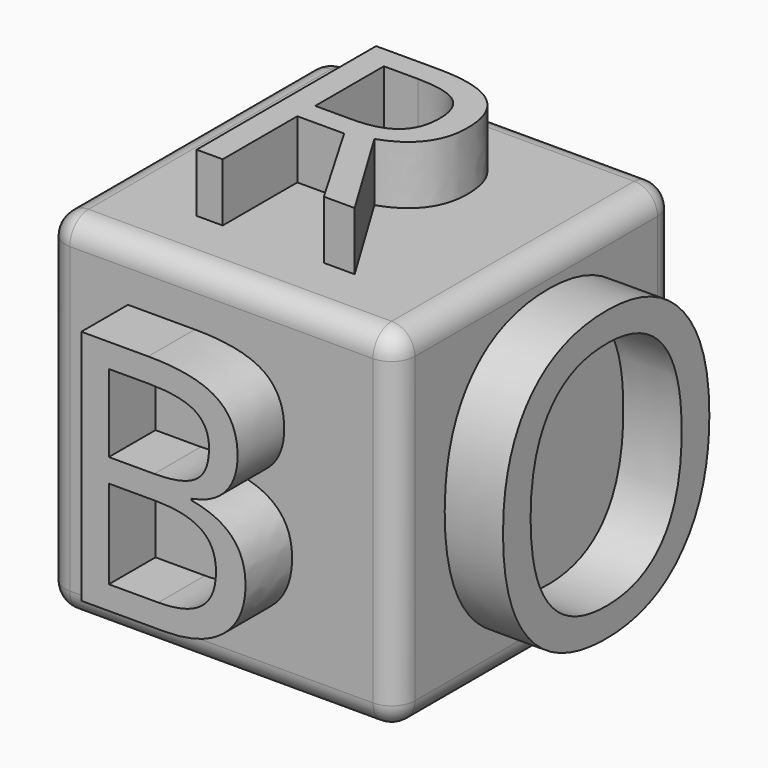
from build123d import *

# Parameters (mm, degrees)
F0_W         = 76.2
F0_H         = 76.2
F1_DEPTH     = 76.2
F2_R         = 5.08
F3_TEXT_SIZE = 68.4524769895
F4_DEPTH     = 12.7
F5_TEXT_SIZE = 85.5601075778
F6_DEPTH     = 12.7
F7_TEXT_SIZE = 72.2860412983
F8_DEPTH     = 12.7


# Not quite as in the source:
# - Text() gives the source's letters only with a copy of the font that has no kerning and outlines rounded to 1/6400 em; it was checked with that copy


with BuildPart() as f1:
    # F0 (on Front) → F1 (new body)
    with BuildSketch(Plane.XZ):
        with Locations((-35.660278523, 38.1)):
            Rectangle(F0_W, F0_H)
    extrude(amount=F1_DEPTH)

    # F2
    f2_edges = [f1.edges().sort_by_distance(p)[0] for p in [
        (-73.760279, -38.1, 76.2),
        (-73.760279, -38.1, 0),
        (-73.760279, 0, 38.1),
        (-73.760279, -76.2, 38.1),
        (2.439721, -38.1, 0),
        (-35.660279, 0, 0),
        (-35.660279, -76.2, 0),
        (2.439721, -76.2, 38.1),
        (-35.660279, -76.2, 76.2),
        (2.439721, -38.1, 76.2),
        (2.439721, 0, 38.1),
        (-35.660279, 0, 76.2),
    ]]
    fillet(f2_edges, radius=F2_R)

    # F3 (on face) → F4 (join)
    with BuildSketch(Plane.XY.offset(76.2)):
        with Locations((-59.5189295709, -61.5189932287)):
            Text('R', F3_TEXT_SIZE, font='Open Sans', text_align=(TextAlign.LEFT, TextAlign.BOTTOM))
    extrude(amount=F4_DEPTH)

    # F5 (on face) → F6 (join)
    with BuildSketch(Plane.YZ.offset(2.439721477)):
        with Locations((-68.2380497456, 7.2336574085)):
            Text('O', F5_TEXT_SIZE, font='Open Sans', text_align=(TextAlign.LEFT, TextAlign.BOTTOM))
    extrude(amount=F6_DEPTH)

    # F7 (on face) → F8 (join)
    with BuildSketch(Plane.XZ.offset(76.2)):
        with Locations((-63.1089471281, 12.463468127)):
            Text('B', F7_TEXT_SIZE, font='Open Sans', text_align=(TextAlign.LEFT, TextAlign.BOTTOM))
    extrude(amount=F8_DEPTH)


solid = f1.part
